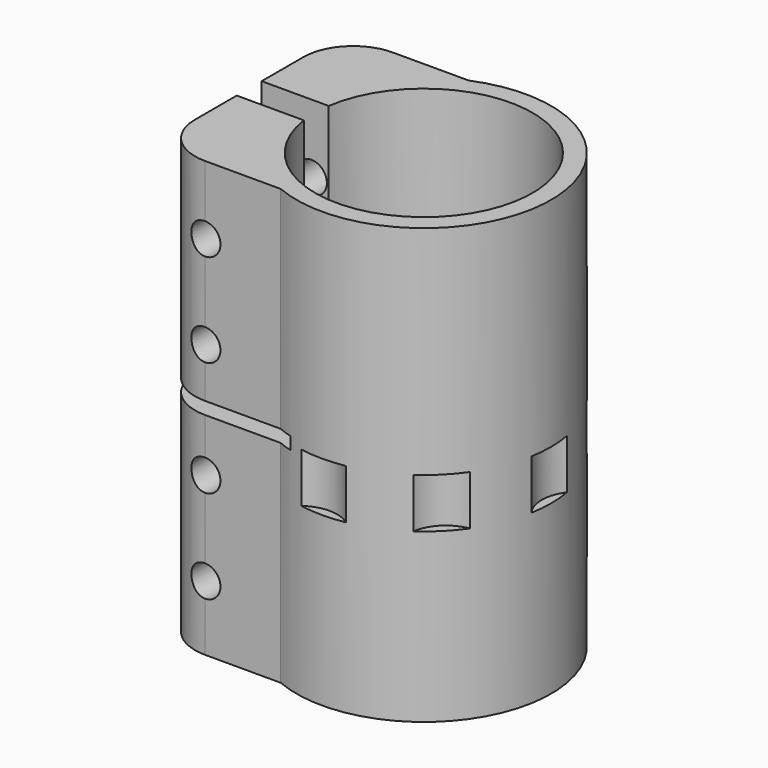
from build123d import *

# Parameters (mm, degrees)
F1_DEPTH       = 35
F3_D           = 5
F3_START       = 1.7550021
F3_CBORE_D     = 10
F3_CBORE_DEPTH = 8
F4_W           = 22.4
F4_H           = 2
F5_DEPTH       = 25
F6_R           = 6
F7_DEPTH       = 8


with BuildPart() as f1:
    # F0 (on Top) → F1 (new body, symmetric)
    with BuildSketch(Plane.XY):
        with BuildLine():
            ThreePointArc((-17.3192642082, 2.5086026559), (17.5, 0), (-17.3192642082, -2.5086026559))
            Line((-17.3192642082, -2.5086026559), (-28.1192642082, -2.5086026559))
            Line((-28.1192642082, -2.5086026559), (-28.1192642082, -10.9086026559))
            ThreePointArc((-28.1192642082, -10.9086026559), (-25.7761184577, -16.5654569054), (-20.1192642082, -18.9086026559))
            Line((-20.1192642082, -18.9086026559), (-7.9192642082, -18.9086026559))
            ThreePointArc((-7.9192642082, -18.9086026559), (20.5, 0), (-7.9192642082, 18.9086026559))
            Line((-7.9192642082, 18.9086026559), (-20.1192642082, 18.9086026559))
            ThreePointArc((-20.1192642082, 18.9086026559), (-25.7761184577, 16.5654569054), (-28.1192642082, 10.9086026559))
            Line((-28.1192642082, 10.9086026559), (-28.1192642082, 2.5086026559))
            Line((-28.1192642082, 2.5086026559), (-17.3192642082, 2.5086026559))
        make_face()
    extrude(amount=F1_DEPTH, both=True)

    # F3 (through all)
    # its depths count from where the whole tool has entered the part; down to there all is cleared
    with Locations(Plane(origin=(0, 18.9086026559, 0), x_dir=(-1, 0, 0), z_dir=(0, 1, 0)).offset(-F3_START)):
        with Locations((20.1192642082, 23.9717778414), (20.1192642082, 8.9717778414), (20.1192642082, -9.5282221586), (20.1192642082, -24.5282221586)):
            CounterBoreHole(F3_D / 2, F3_CBORE_D / 2, F3_CBORE_DEPTH)

    # F4 (on Front) → F5 (cut, symmetric)
    with BuildSketch(Plane.XZ):
        with Locations((-16.9192642082, -0.0041035237)):
            Rectangle(F4_W, F4_H)
    extrude(amount=F5_DEPTH, both=True, mode=Mode.SUBTRACT)

    # F6 (on Top) → F7 (cut)
    with BuildSketch(Plane.XY):
        with Locations((0, -25)):
            Circle(F6_R)
        with Locations((17.6776695297, -17.6776695297)):
            Circle(F6_R)
        with Locations((25, 0)):
            Circle(F6_R)
        with Locations((17.6776695297, 17.6776695297)):
            Circle(F6_R)
        with Locations((0, 25)):
            Circle(F6_R)
    extrude(amount=-F7_DEPTH, mode=Mode.SUBTRACT)


solid = f1.part
